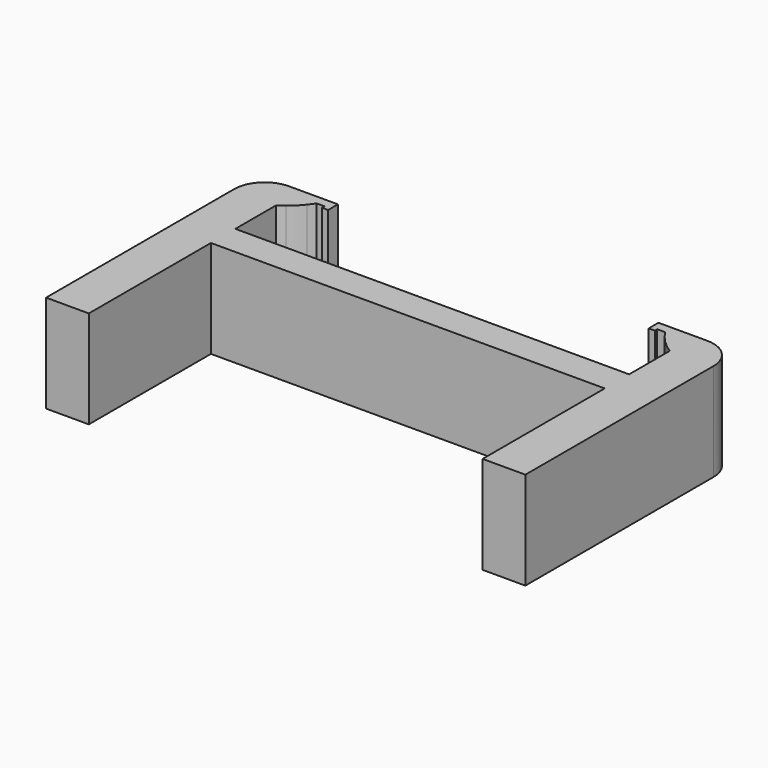
from build123d import *

# Parameters (mm, degrees)
F0_W     = 1
F0_H     = 0.5
F1_DEPTH = 16
F2_R     = 5


with BuildPart() as f1:
    # F0 (on Top) → F1 (new body)
    with BuildSketch(Plane.XY):
        Polygon((32.25, -2.5), (32.25, 2.5), (28.25, 2.5), (-28.25, 2.5), (-32.25, 2.5), (-32.25, -2.5), align=None)
        Polygon((32.25, 10.8), (32.25, 2.5), (32.25, -2.5), (32.25, -27.5), (39.25, -27.5), (39.25, 14.5), (32.25, 14.5), align=None)
        with BuildLine():
            ThreePointArc((28.55, 14.5), (30.1958719271, 12.4458719271), (32.25, 10.8))
            Line((32.25, 10.8), (32.25, 14.5))
            Line((32.25, 14.5), (28.55, 14.5))
        make_face()
        Polygon((27.25, 14.5), (28.25, 14.5), (28.55, 14.5), (32.25, 14.5), (39.25, 14.5), (39.25, 16), (26.25, 16), (26.25, 14.5), align=None)
        Polygon((-32.25, -27.5), (-32.25, -2.5), (-32.25, 2.5), (-39.25, 2.5), (-39.25, -27.5), align=None)
        Polygon((-39.25, 2.5), (-32.25, 2.5), (-32.25, 10.5), (-32.25, 10.8), (-32.25, 14.5), (-39.25, 14.5), align=None)
        with Locations((26.75, 14.25)):
            Rectangle(F0_W, F0_H)
        Polygon((-28.55, 14.5), (-28.25, 14.5), (-27.25, 14.5), (-26.25, 14.5), (-26.25, 16), (-39.25, 16), (-39.25, 14.5), (-32.25, 14.5), align=None)
        with BuildLine():
            Line((-32.25, 14.5), (-32.25, 10.8))
            ThreePointArc((-32.25, 10.8), (-31.7185283382, 11.1576250938), (-31.2068981187, 11.5431018813))
            Line((-31.2068981187, 11.5431018813), (-29.2931018813, 13.4568981187))
            ThreePointArc((-29.2931018813, 13.4568981187), (-28.9076250938, 13.9685283382), (-28.55, 14.5))
            Line((-28.55, 14.5), (-32.25, 14.5))
        make_face()
        with Locations((-26.75, 14.25)):
            Rectangle(F0_W, F0_H)
        with BuildLine():
            Line((-29.2931018813, 13.4568981187), (-31.2068981187, 11.5431018813))
            ThreePointArc((-31.2068981187, 11.5431018813), (-30.1958719271, 12.4458719271), (-29.2931018813, 13.4568981187))
        make_face()
    extrude(amount=F1_DEPTH)

    # F2
    f2_edges = [f1.edges().sort_by_distance(p)[0] for p in [
        (-39.25, 16, 8),
        (39.25, 16, 8),
    ]]
    fillet(f2_edges, radius=F2_R)


solid = f1.part
